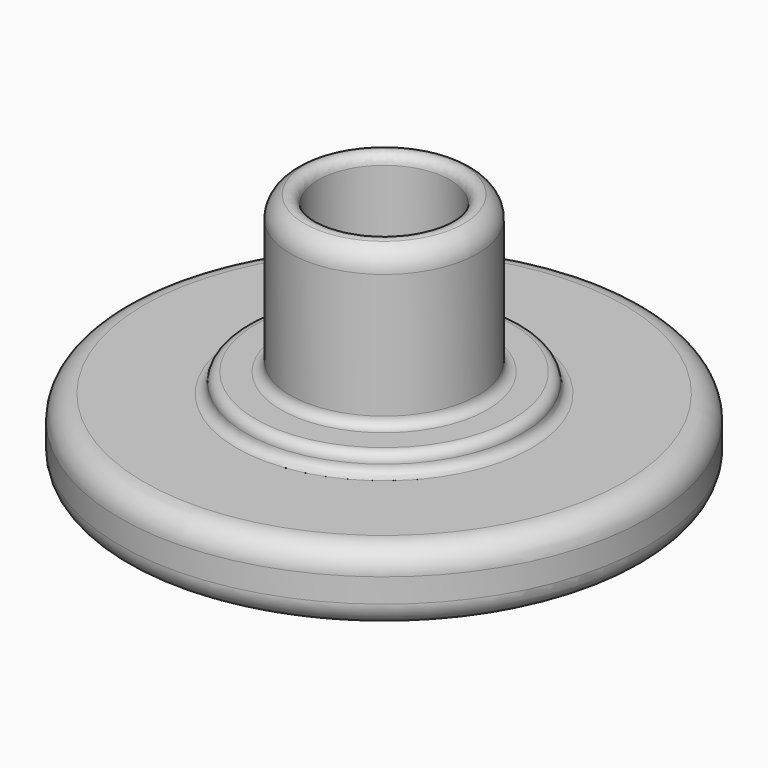
from build123d import *

# Parameters (mm, degrees)
F0_R      = 11
F1_DEPTH  = 3
F2_R      = 5.75
F3_DEPTH  = 0.8
F4_R      = 3.9
F4_R_2    = 2.75
F5_DEPTH  = 6.6
F8_R      = 2.4
F8_R_2    = 2
F9_DEPTH  = 0.6
F6_R      = 1.2
F10_DEPTH = 7
F11_R     = 1
F12_R     = 0.39999


# Not quite as in the source:
# - a fillet or chamfer is up to 0.001 mm smaller than in the source, because OpenCascade refuses the exact size


with BuildPart() as f1:
    # F0 (on Top) → F1 (new body)
    with BuildSketch(Plane.XY):
        Circle(F0_R)
    extrude(amount=F1_DEPTH)

    # F2 (on face) → F3 (join)
    with BuildSketch(Plane.XY.offset(3)):
        Circle(F2_R)
    extrude(amount=F3_DEPTH)

    # F4 (on face) → F5 (join)
    with BuildSketch(Plane.XY.offset(3.8)):
        Circle(F4_R)
        Circle(F4_R_2, mode=Mode.SUBTRACT)
    extrude(amount=F5_DEPTH)

    # F8 (on offset) → F9 (cut)
    with BuildSketch(Plane.XY.offset(4.8)):
        Circle(F8_R)
        Circle(F8_R_2, mode=Mode.SUBTRACT)
    extrude(amount=F9_DEPTH, mode=Mode.SUBTRACT)

    # F6 (on face) → F10 (cut)
    with BuildSketch(Plane.XY.offset(10.4)):
        Circle(F6_R)
    extrude(amount=-F10_DEPTH, mode=Mode.SUBTRACT)

    # F11
    f11_edges = [f1.edges().sort_by_distance(p)[0] for p in [
        (-11, 0, 3),
        (-11, 0, 0),
        (-3.9, 0, 10.4),
    ]]
    fillet(f11_edges, radius=F11_R)

    # F12 (radius 0.4 in the source; OpenCascade refuses exactly that, so slightly less here)
    f12_edges = [f1.edges().sort_by_distance(p)[0] for p in [
        (-5.75, 0, 3.8),
        (-3.9, 0, 3.8),
        (-2.9, 0, 10.4),
        (-2.75, 0, 10.4),
        (-2.75, 0, 3.8),
        (-5.75, 0, 3),
    ]]
    fillet(f12_edges, radius=F12_R)


solid = f1.part
